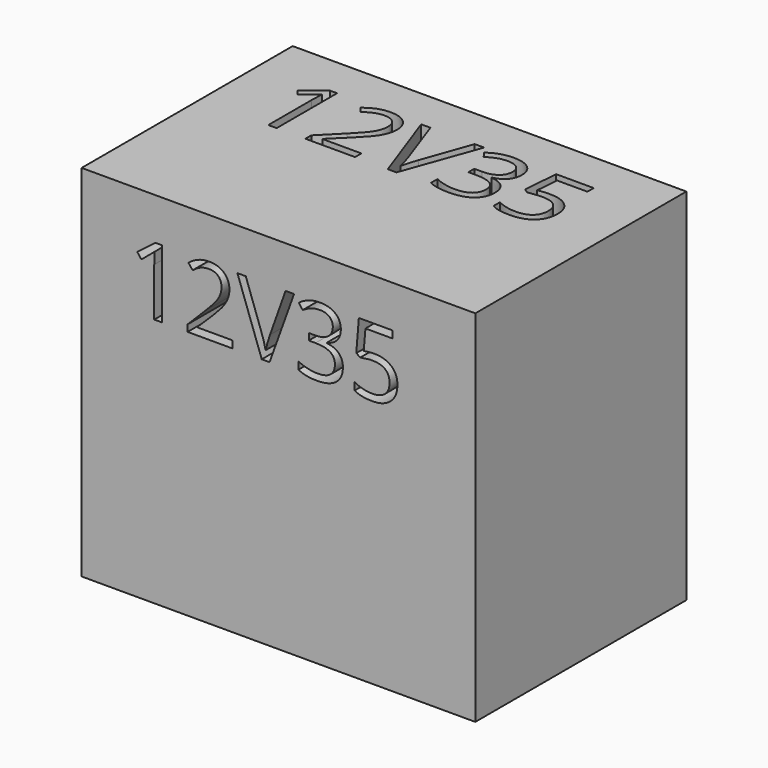
from build123d import *

# Parameters (mm, degrees)
F0_W         = 197
F0_H         = 132
F1_DEPTH     = 180
F2_TEXT_SIZE = 52.9516414122
F3_DEPTH     = 25
F4_TEXT_SIZE = 47.6338797145
F5_DEPTH     = 25


# Not quite as in the source:
# - Text() gives the source's letters only with a copy of the font that has no kerning and outlines rounded to 1/6400 em; it was checked with that copy


with BuildPart() as f1:
    # F0 (on Top) → F1 (new body)
    with BuildSketch(Plane.XY):
        with Locations((98.5, 66)):
            Rectangle(F0_W, F0_H)
    extrude(amount=F1_DEPTH)

    # F2 (on face) → F3 (cut)
    with BuildSketch(Plane.XY.offset(180)):
        with Locations((20, 73.8748181832)):
            Text('12V35', F2_TEXT_SIZE, font='Open Sans', text_align=(TextAlign.LEFT, TextAlign.BOTTOM))
    extrude(amount=-F3_DEPTH, mode=Mode.SUBTRACT)

    # F4 (on face) → F5 (cut)
    with BuildSketch(Plane.XZ):
        with Locations((23.4696939588, 124.9946504831)):
            Text('12V35', F4_TEXT_SIZE, font='Open Sans', text_align=(TextAlign.LEFT, TextAlign.BOTTOM))
    extrude(amount=-F5_DEPTH, mode=Mode.SUBTRACT)


solid = f1.part
